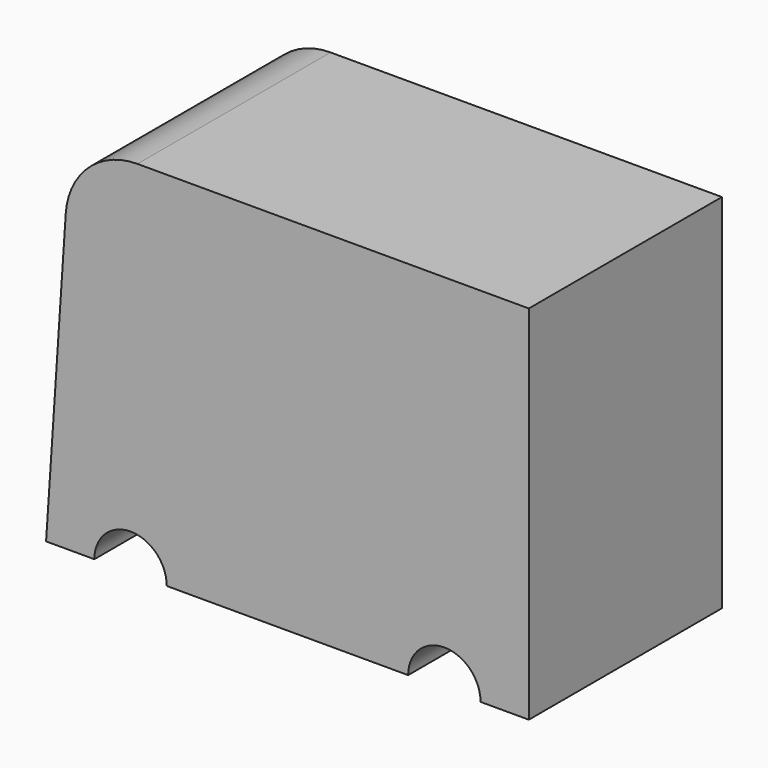
from build123d import *

# Parameters (mm, degrees)
F0_W     = 101.6
F0_H     = 50.8
F1_DEPTH = 76.2
F3_DEPTH = 50.8
F4_W     = 81.28
F4_H     = 10.16
F5_DEPTH = 3.302
F6_R     = 1.27
F7_DEPTH = 10.16
F8_SIZE2 = 76.19999
F8_SIZE  = 5.07999
F9_R     = 15.1271850899


# Not quite as in the source:
# - a fillet or chamfer is up to 0.001 mm smaller than in the source, because OpenCascade refuses the exact size


with BuildPart() as f1:
    # F0 (on Top) → F1 (new body)
    with BuildSketch(Plane.XY):
        with Locations((30.5125243939, 8.8571563035)):
            Rectangle(F0_W, F0_H)
    extrude(amount=F1_DEPTH)

    # F2 (on face) → F3 (cut)
    with BuildSketch(Plane.XZ.offset(16.5428436965)):
        with BuildLine():
            Line((-2.5074756061, 0), (5.1125243939, 0))
            ThreePointArc((5.1125243939, 0), (-2.5074756061, 7.62), (-10.1274756061, 0))
            Line((-10.1274756061, 0), (-2.5074756061, 0))
        make_face()
        with BuildLine():
            Line((63.5325243939, 0), (71.1525243939, 0))
            ThreePointArc((71.1525243939, 0), (63.5325243939, 7.62), (55.9125243939, 0))
            Line((55.9125243939, 0), (63.5325243939, 0))
        make_face()
    extrude(amount=-F3_DEPTH, mode=Mode.SUBTRACT)

    # F8 (size 5.08 and 76.2 in the source; OpenCascade refuses exactly that, so slightly less here)
    f8_edges = [f1.edges().sort_by_distance(p)[0] for p in [
        (-20.287476, 8.857156, 76.2),
    ]]
    f8_side = f1.faces().sort_by_distance((30.512524, 8.857156, 76.2))[0]
    chamfer(f8_edges, length=F8_SIZE, length2=F8_SIZE2, reference=f8_side)

    # F9
    f9_edges = [f1.edges().sort_by_distance(p)[0] for p in [
        (-15.207486, 8.857156, 76.2),
    ]]
    fillet(f9_edges, radius=F9_R)


with BuildPart() as f5:
    # F4 (on face) → F5 (new body)
    with BuildSketch(Plane(origin=(0, 0, 0), x_dir=(1, 0, 0), z_dir=(0, 0, -1))):
        with Locations((30.5125243939, -8.8571563035)):
            Rectangle(F4_W, F4_H)
    extrude(amount=F5_DEPTH)

    # F6 (on face) → F7 (cut)
    with BuildSketch(Plane(origin=(0, 13.9371563035, 0), x_dir=(-1, 0, 0), z_dir=(0, 1, 0))):
        with Locations((-63.5325243939, 0)):
            Circle(F6_R)
        with Locations((2.5074756061, 0)):
            Circle(F6_R)
    extrude(amount=-F7_DEPTH, mode=Mode.SUBTRACT)


solid = Compound([f1.part, f5.part])
